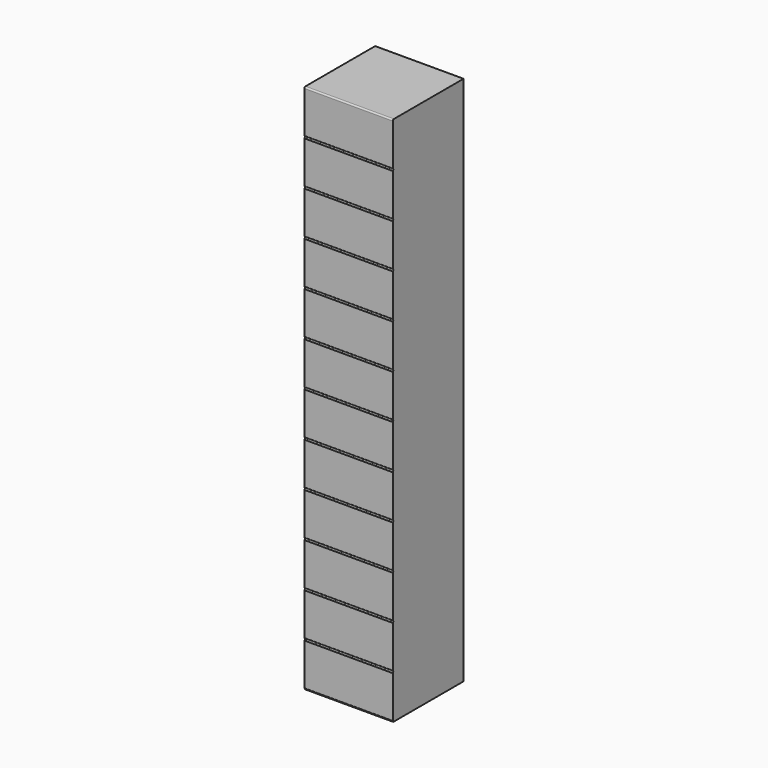
from build123d import *

# Parameters (mm, degrees)
F0_W        = 20
F0_H        = 20
F1_DEPTH    = 120
F3_DEPTH    = 0.125
F4_T1_DEPTH = 20
F4_T3_DEPTH = 21.5625


# Not quite as in the source:
# - a fillet or chamfer that OpenCascade refuses, or shapes differently, is made with other operations: its cross-section is extruded or revolved along the edge and cut away or added


with BuildPart() as f1:
    # F0 (on Top) → F1 (new body)
    with BuildSketch(Plane.XY):
        Rectangle(F0_W, F0_H)
    extrude(amount=F1_DEPTH)

    # F2 (on face) → F3 (cut)
    with BuildSketch(Plane.XZ.offset(10)):
        with BuildLine():
            ThreePointArc((-10, 110.25), (-10.25, 110), (-10, 109.75))
            Line((-10, 109.75), (10, 109.75))
            ThreePointArc((10, 109.75), (10.25, 110), (10, 110.25))
            Line((10, 110.25), (-10, 110.25))
        make_face()
        with BuildLine():
            ThreePointArc((-10, 0.25), (-10.25, 0), (-10, -0.25))
            Line((-10, -0.25), (15, -0.25))
            ThreePointArc((15, -0.25), (15.25, 0), (15, 0.25))
            Line((15, 0.25), (-10, 0.25))
        make_face()
        with BuildLine():
            ThreePointArc((-10, 10.25), (-10.25, 10), (-10, 9.75))
            Line((-10, 9.75), (10, 9.75))
            ThreePointArc((10, 9.75), (10.25, 10), (10, 10.25))
            Line((10, 10.25), (-10, 10.25))
        make_face()
        with BuildLine():
            ThreePointArc((-10, 20.25), (-10.25, 20), (-10, 19.75))
            Line((-10, 19.75), (10, 19.75))
            ThreePointArc((10, 19.75), (10.25, 20), (10, 20.25))
            Line((10, 20.25), (-10, 20.25))
        make_face()
        with BuildLine():
            ThreePointArc((-10, 30.25), (-10.25, 30), (-10, 29.75))
            Line((-10, 29.75), (10, 29.75))
            ThreePointArc((10, 29.75), (10.25, 30), (10, 30.25))
            Line((10, 30.25), (-10, 30.25))
        make_face()
        with BuildLine():
            ThreePointArc((-10, 40.25), (-10.25, 40), (-10, 39.75))
            Line((-10, 39.75), (10, 39.75))
            ThreePointArc((10, 39.75), (10.25, 40), (10, 40.25))
            Line((10, 40.25), (-10, 40.25))
        make_face()
        with BuildLine():
            ThreePointArc((-10, 50.25), (-10.25, 50), (-10, 49.75))
            Line((-10, 49.75), (10, 49.75))
            ThreePointArc((10, 49.75), (10.25, 50), (10, 50.25))
            Line((10, 50.25), (-10, 50.25))
        make_face()
        with BuildLine():
            ThreePointArc((-10, 60.25), (-10.25, 60), (-10, 59.75))
            Line((-10, 59.75), (10, 59.75))
            ThreePointArc((10, 59.75), (10.25, 60), (10, 60.25))
            Line((10, 60.25), (-10, 60.25))
        make_face()
        with BuildLine():
            ThreePointArc((-10, 70.25), (-10.25, 70), (-10, 69.75))
            Line((-10, 69.75), (10, 69.75))
            ThreePointArc((10, 69.75), (10.25, 70), (10, 70.25))
            Line((10, 70.25), (-10, 70.25))
        make_face()
        with BuildLine():
            ThreePointArc((-10, 80.25), (-10.25, 80), (-10, 79.75))
            Line((-10, 79.75), (10, 79.75))
            ThreePointArc((10, 79.75), (10.25, 80), (10, 80.25))
            Line((10, 80.25), (-10, 80.25))
        make_face()
        with BuildLine():
            ThreePointArc((-10, 90.25), (-10.25, 90), (-10, 89.75))
            Line((-10, 89.75), (10, 89.75))
            ThreePointArc((10, 89.75), (10.25, 90), (10, 90.25))
            Line((10, 90.25), (-10, 90.25))
        make_face()
        with BuildLine():
            ThreePointArc((-10, 100.25), (-10.25, 100), (-10, 99.75))
            Line((-10, 99.75), (10, 99.75))
            ThreePointArc((10, 99.75), (10.25, 100), (10, 100.25))
            Line((10, 100.25), (-10, 100.25))
        make_face()
    extrude(amount=-F3_DEPTH, mode=Mode.SUBTRACT)

    # F4: fillet of radius 0.3125 on 24 edges, made by hand

    # F4_s2 → F4_t1 (join)
    with BuildSketch(Plane.YZ.offset(-10)):
        with BuildLine():
            ThreePointArc((-9.875, 60), (-9.9079915028, 59.8602457514), (-10, 59.75))
            Line((-10, 59.75), (-9.875, 59.75))
            Line((-9.875, 59.75), (-9.875, 60))
        make_face()
        with BuildLine():
            ThreePointArc((-10, 60.25), (-9.9079915028, 60.1397542486), (-9.875, 60))
            Line((-9.875, 60), (-9.875, 60.25))
            Line((-9.875, 60.25), (-10, 60.25))
        make_face()
        with BuildLine():
            ThreePointArc((-10, 0.25), (-9.9079915028, 0.1397542486), (-9.875, 0))
            Line((-9.875, 0), (-9.875, 0.25))
            Line((-9.875, 0.25), (-10, 0.25))
        make_face()
        with BuildLine():
            ThreePointArc((-10, 9.75), (-9.9079915028, 9.8602457514), (-9.875, 10))
            Line((-9.875, 10), (-9.875, 9.75))
            Line((-9.875, 9.75), (-10, 9.75))
        make_face()
        with BuildLine():
            ThreePointArc((-10, 10.25), (-9.9079915028, 10.1397542486), (-9.875, 10))
            Line((-9.875, 10), (-9.875, 10.25))
            Line((-9.875, 10.25), (-10, 10.25))
        make_face()
        with BuildLine():
            ThreePointArc((-10, 20.25), (-9.9079915028, 20.1397542486), (-9.875, 20))
            Line((-9.875, 20), (-9.875, 20.25))
            Line((-9.875, 20.25), (-10, 20.25))
        make_face()
        with BuildLine():
            ThreePointArc((-9.875, 20), (-9.9079915028, 19.8602457514), (-10, 19.75))
            Line((-10, 19.75), (-9.875, 19.75))
            Line((-9.875, 19.75), (-9.875, 20))
        make_face()
        with BuildLine():
            ThreePointArc((-9.875, 30), (-9.9079915028, 29.8602457514), (-10, 29.75))
            Line((-10, 29.75), (-9.875, 29.75))
            Line((-9.875, 29.75), (-9.875, 30))
        make_face()
        with BuildLine():
            ThreePointArc((-10, 30.25), (-9.9079915028, 30.1397542486), (-9.875, 30))
            Line((-9.875, 30), (-9.875, 30.25))
            Line((-9.875, 30.25), (-10, 30.25))
        make_face()
        with BuildLine():
            ThreePointArc((-10, 40.25), (-9.9079915028, 40.1397542486), (-9.875, 40))
            Line((-9.875, 40), (-9.875, 40.25))
            Line((-9.875, 40.25), (-10, 40.25))
        make_face()
        with BuildLine():
            ThreePointArc((-9.875, 40), (-9.9079915028, 39.8602457514), (-10, 39.75))
            Line((-10, 39.75), (-9.875, 39.75))
            Line((-9.875, 39.75), (-9.875, 40))
        make_face()
        with BuildLine():
            ThreePointArc((-9.875, 50), (-9.9079915028, 49.8602457514), (-10, 49.75))
            Line((-10, 49.75), (-9.875, 49.75))
            Line((-9.875, 49.75), (-9.875, 50))
        make_face()
        with BuildLine():
            ThreePointArc((-10, 50.25), (-9.9079915028, 50.1397542486), (-9.875, 50))
            Line((-9.875, 50), (-9.875, 50.25))
            Line((-9.875, 50.25), (-10, 50.25))
        make_face()
        with BuildLine():
            ThreePointArc((-10, 70.25), (-9.9079915028, 70.1397542486), (-9.875, 70))
            Line((-9.875, 70), (-9.875, 70.25))
            Line((-9.875, 70.25), (-10, 70.25))
        make_face()
        with BuildLine():
            ThreePointArc((-9.875, 70), (-9.9079915028, 69.8602457514), (-10, 69.75))
            Line((-10, 69.75), (-9.875, 69.75))
            Line((-9.875, 69.75), (-9.875, 70))
        make_face()
        with BuildLine():
            ThreePointArc((-9.875, 80), (-9.9079915028, 79.8602457514), (-10, 79.75))
            Line((-10, 79.75), (-9.875, 79.75))
            Line((-9.875, 79.75), (-9.875, 80))
        make_face()
        with BuildLine():
            ThreePointArc((-10, 80.25), (-9.9079915028, 80.1397542486), (-9.875, 80))
            Line((-9.875, 80), (-9.875, 80.25))
            Line((-9.875, 80.25), (-10, 80.25))
        make_face()
        with BuildLine():
            ThreePointArc((-10, 90.25), (-9.9079915028, 90.1397542486), (-9.875, 90))
            Line((-9.875, 90), (-9.875, 90.25))
            Line((-9.875, 90.25), (-10, 90.25))
        make_face()
        with BuildLine():
            ThreePointArc((-9.875, 90), (-9.9079915028, 89.8602457514), (-10, 89.75))
            Line((-10, 89.75), (-9.875, 89.75))
            Line((-9.875, 89.75), (-9.875, 90))
        make_face()
        with BuildLine():
            ThreePointArc((-10, 100.25), (-9.9079915028, 100.1397542486), (-9.875, 100))
            Line((-9.875, 100), (-9.875, 100.25))
            Line((-9.875, 100.25), (-10, 100.25))
        make_face()
        with BuildLine():
            ThreePointArc((-9.875, 100), (-9.9079915028, 99.8602457514), (-10, 99.75))
            Line((-10, 99.75), (-9.875, 99.75))
            Line((-9.875, 99.75), (-9.875, 100))
        make_face()
        with BuildLine():
            ThreePointArc((-9.875, 110), (-9.9079915028, 109.8602457514), (-10, 109.75))
            Line((-10, 109.75), (-9.875, 109.75))
            Line((-9.875, 109.75), (-9.875, 110))
        make_face()
        with BuildLine():
            ThreePointArc((-10, 110.25), (-9.9079915028, 110.1397542486), (-9.875, 110))
            Line((-9.875, 110), (-9.875, 110.25))
            Line((-9.875, 110.25), (-10, 110.25))
        make_face()
    extrude(amount=F4_T1_DEPTH)

    # F4_s4 → F4_t3 (cut)
    with BuildSketch(Plane.YZ.offset(-10.78125)):
        with BuildLine():
            ThreePointArc((-10, 119.6875), (-9.9084708691, 119.9084708691), (-9.6875, 120))
            Line((-9.6875, 120), (-10, 120))
            Line((-10, 120), (-10, 119.6875))
        make_face()
    extrude(amount=F4_T3_DEPTH, mode=Mode.SUBTRACT)


solid = f1.part
